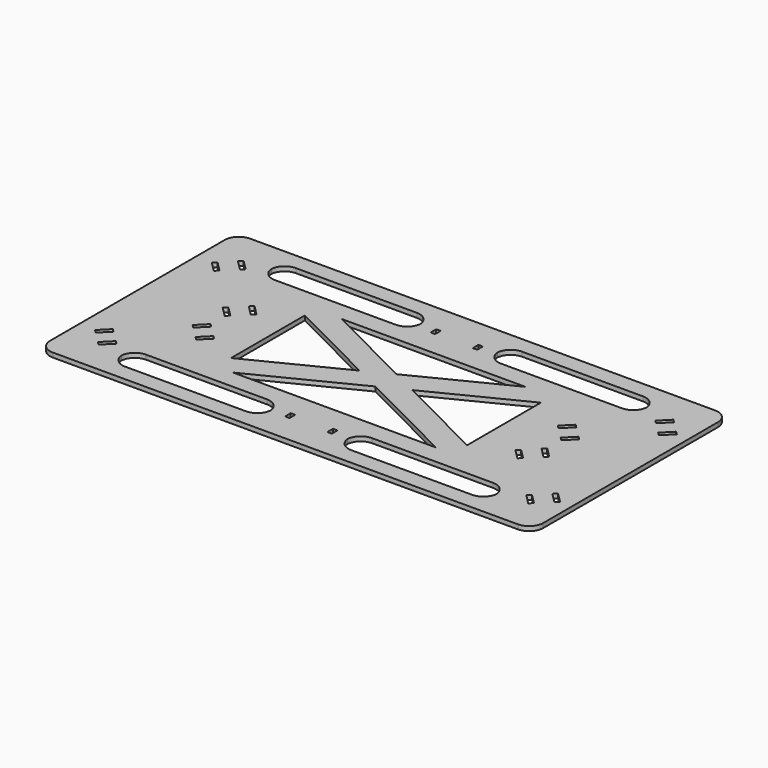
from build123d import *

# Parameters (mm, degrees)
F0_W        = 350
F0_H        = 175
F0_W_2      = 3.175
F0_H_2      = 5
F1_DEPTH    = 3.175
F3_DEPTH    = 25
F4_W        = 105.779197067
F4_H        = 18.4744439814
F5_DEPTH    = 25
F6_T1_DEPTH = 3.175
F6_T3_DEPTH = 53.175
F8_DEPTH    = 25


# Not quite as in the source:
# - a fillet or chamfer that OpenCascade refuses, or shapes differently, is made with other operations: its cross-section is extruded or revolved along the edge and cut away or added


with BuildPart() as f1:
    # F0 (on Top) → F1 (new body)
    with BuildSketch(Plane.XY):
        Rectangle(F0_W, F0_H)
        with Locations((-15, -64.5)):
            Rectangle(F0_W_2, F0_H_2, mode=Mode.SUBTRACT)
        with Locations((15.001, -64.5)):
            Rectangle(F0_W_2, F0_H_2, mode=Mode.SUBTRACT)
        with Locations((-15, 64.5)):
            Rectangle(F0_W_2, F0_H_2, mode=Mode.SUBTRACT)
        with Locations((15.001, 64.5)):
            Rectangle(F0_W_2, F0_H_2, mode=Mode.SUBTRACT)
    extrude(amount=F1_DEPTH)

    # F2 (on face) → F3 (cut)
    with BuildSketch(Plane.XY.offset(3.175)):
        Polygon((-156.5389321881, -44.7351793874), (-163.61, -51.8062471993), (-161.3649359697, -54.0513112295), (-154.2938681579, -46.9802434177), align=None)
        Polygon((-146.2837625406, -54.9903490349), (-153.3548303525, -62.0614168468), (-151.1097663222, -64.3064808771), (-144.0386985103, -57.2354130652), align=None)
        Polygon((159.2439321881, 44.7353613385), (166.315, 51.8064291503), (164.0699359697, 54.0514931806), (156.9988681579, 46.9804253687), align=None)
        Polygon((148.9887625406, 54.990530986), (156.0598303525, 62.0615987979), (153.8147663222, 64.3066628282), (146.7436985103, 57.2355950163), align=None)
        Polygon((-161.3649359697, 54.0513112295), (-163.61, 51.8062471993), (-156.5389321881, 44.7351793874), (-154.2938681579, 46.9802434177), align=None)
        Polygon((-151.0729967696, 64.3432504297), (-153.3180607998, 62.0981863994), (-146.246992988, 55.0271185876), (-144.0019289577, 57.2721826178), align=None)
        Polygon((157.0488681579, -46.9683818087), (164.1199359697, -54.0394496205), (166.365, -51.7943855903), (159.2939321881, -44.7233177784), align=None)
        Polygon((146.7569289577, -57.2603210088), (153.8279967696, -64.3313888207), (156.0730607998, -62.0863247904), (149.001992988, -55.0152569786), align=None)
        Polygon((118.5822592613, -8.5017729121), (125.6533270732, -15.572840724), (127.8983911035, -13.3277766937), (120.8273232916, -6.2567088818), align=None)
        Polygon((108.2903200611, -18.7937121123), (115.361387873, -25.8647799241), (117.6064519033, -23.6197158939), (110.5353840914, -16.548648082), align=None)
        Polygon((120.7773232916, 6.2687524419), (127.8483911035, 13.3398202538), (125.6033270732, 15.5848842841), (118.5322592613, 8.5138164722), align=None)
        Polygon((110.522153644, 16.5239220895), (117.5932214559, 23.5949899013), (115.3481574256, 25.8400539316), (108.2770896138, 18.7689861197), align=None)
        Polygon((-122.8983270732, 15.584702333), (-125.1433911035, 13.3396383027), (-118.0723232916, 6.2685704909), (-115.8272592613, 8.5136345211), align=None)
        Polygon((-112.606387873, 25.8766415332), (-114.8514519033, 23.6315775029), (-107.7803840914, 16.560509691), (-105.5353200611, 18.8055737213), align=None)
        Polygon((-118.0723232916, -6.2685704909), (-125.1433911035, -13.3396383027), (-122.8983270732, -15.584702333), (-115.8272592613, -8.5136345211), align=None)
        Polygon((-107.817153644, -16.5237401384), (-114.8882214559, -23.5948079503), (-112.6431574256, -25.8398719805), (-105.5720896138, -18.7688041687), align=None)
    extrude(amount=-F3_DEPTH, mode=Mode.SUBTRACT)

    # F4 (on face) → F5 (cut)
    with BuildSketch(Plane.XY.offset(3.175)):
        with Locations((-80.2089292556, 66.4726350559)):
            Rectangle(F4_W, F4_H)
        with Locations((-80.2089292556, -66.4726350559)):
            Rectangle(F4_W, F4_H)
        with Locations((80.2089292556, -66.4726350559)):
            Rectangle(F4_W, F4_H)
        with Locations((80.2089292556, 66.4726350559)):
            Rectangle(F4_W, F4_H)
    extrude(amount=-F5_DEPTH, mode=Mode.SUBTRACT)

    # F6: fillet of radius 10 on 20 edges, made by hand

    # F6_s2 → F6_t1 (join)
    with BuildSketch(Plane.XY):
        with BuildLine():
            ThreePointArc((-133.0985277891, -65.7098570466), (-130.169595601, -72.7809248585), (-123.0985277891, -75.7098570466))
            Line((-123.0985277891, -75.7098570466), (-133.0985277891, -75.7098570466))
            Line((-133.0985277891, -75.7098570466), (-133.0985277891, -65.7098570466))
        make_face()
        with BuildLine():
            ThreePointArc((-123.0985277891, -57.2354130652), (-130.169595601, -60.1643452533), (-133.0985277891, -67.2354130652))
            Line((-133.0985277891, -67.2354130652), (-133.0985277891, -57.2354130652))
            Line((-133.0985277891, -57.2354130652), (-123.0985277891, -57.2354130652))
        make_face()
        with BuildLine():
            ThreePointArc((-37.3193307221, -57.2354130652), (-30.2482629102, -60.1643452533), (-27.3193307221, -67.2354130652))
            Line((-27.3193307221, -67.2354130652), (-27.3193307221, -57.2354130652))
            Line((-27.3193307221, -57.2354130652), (-37.3193307221, -57.2354130652))
        make_face()
        with BuildLine():
            ThreePointArc((-37.3193307221, -75.7098570466), (-30.2482629102, -72.7809248585), (-27.3193307221, -65.7098570466))
            Line((-27.3193307221, -65.7098570466), (-27.3193307221, -75.7098570466))
            Line((-27.3193307221, -75.7098570466), (-37.3193307221, -75.7098570466))
        make_face()
        with BuildLine():
            ThreePointArc((123.0985277891, -57.2354130652), (130.169595601, -60.1643452533), (133.0985277891, -67.2354130652))
            Line((133.0985277891, -67.2354130652), (133.0985277891, -57.2354130652))
            Line((133.0985277891, -57.2354130652), (123.0985277891, -57.2354130652))
        make_face()
        with BuildLine():
            ThreePointArc((123.0985277891, -75.7098570466), (130.169595601, -72.7809248585), (133.0985277891, -65.7098570466))
            Line((133.0985277891, -65.7098570466), (133.0985277891, -75.7098570466))
            Line((133.0985277891, -75.7098570466), (123.0985277891, -75.7098570466))
        make_face()
        with BuildLine():
            ThreePointArc((37.3193307221, -57.2354130652), (30.2482629102, -60.1643452533), (27.3193307221, -67.2354130652))
            Line((27.3193307221, -67.2354130652), (27.3193307221, -57.2354130652))
            Line((27.3193307221, -57.2354130652), (37.3193307221, -57.2354130652))
        make_face()
        with BuildLine():
            ThreePointArc((27.3193307221, -65.7098570466), (30.2482629102, -72.7809248585), (37.3193307221, -75.7098570466))
            Line((37.3193307221, -75.7098570466), (27.3193307221, -75.7098570466))
            Line((27.3193307221, -75.7098570466), (27.3193307221, -65.7098570466))
        make_face()
        with BuildLine():
            ThreePointArc((133.0985277891, 65.7098570466), (130.169595601, 72.7809248585), (123.0985277891, 75.7098570466))
            Line((123.0985277891, 75.7098570466), (133.0985277891, 75.7098570466))
            Line((133.0985277891, 75.7098570466), (133.0985277891, 65.7098570466))
        make_face()
        with BuildLine():
            ThreePointArc((133.0985277891, 67.2354130652), (130.169595601, 60.1643452533), (123.0985277891, 57.2354130652))
            Line((123.0985277891, 57.2354130652), (133.0985277891, 57.2354130652))
            Line((133.0985277891, 57.2354130652), (133.0985277891, 67.2354130652))
        make_face()
        with BuildLine():
            ThreePointArc((37.3193307221, 75.7098570466), (30.2482629102, 72.7809248585), (27.3193307221, 65.7098570466))
            Line((27.3193307221, 65.7098570466), (27.3193307221, 75.7098570466))
            Line((27.3193307221, 75.7098570466), (37.3193307221, 75.7098570466))
        make_face()
        with BuildLine():
            ThreePointArc((27.3193307221, 67.2354130652), (30.2482629102, 60.1643452533), (37.3193307221, 57.2354130652))
            Line((37.3193307221, 57.2354130652), (27.3193307221, 57.2354130652))
            Line((27.3193307221, 57.2354130652), (27.3193307221, 67.2354130652))
        make_face()
        with BuildLine():
            ThreePointArc((-27.3193307221, 65.7098570466), (-30.2482629102, 72.7809248585), (-37.3193307221, 75.7098570466))
            Line((-37.3193307221, 75.7098570466), (-27.3193307221, 75.7098570466))
            Line((-27.3193307221, 75.7098570466), (-27.3193307221, 65.7098570466))
        make_face()
        with BuildLine():
            ThreePointArc((-37.3193307221, 57.2354130652), (-30.2482629102, 60.1643452533), (-27.3193307221, 67.2354130652))
            Line((-27.3193307221, 67.2354130652), (-27.3193307221, 57.2354130652))
            Line((-27.3193307221, 57.2354130652), (-37.3193307221, 57.2354130652))
        make_face()
        with BuildLine():
            ThreePointArc((-133.0985277891, 67.2354130652), (-130.169595601, 60.1643452533), (-123.0985277891, 57.2354130652))
            Line((-123.0985277891, 57.2354130652), (-133.0985277891, 57.2354130652))
            Line((-133.0985277891, 57.2354130652), (-133.0985277891, 67.2354130652))
        make_face()
        with BuildLine():
            ThreePointArc((-133.0985277891, 65.7098570466), (-130.169595601, 72.7809248585), (-123.0985277891, 75.7098570466))
            Line((-123.0985277891, 75.7098570466), (-133.0985277891, 75.7098570466))
            Line((-133.0985277891, 75.7098570466), (-133.0985277891, 65.7098570466))
        make_face()
    extrude(amount=F6_T1_DEPTH)

    # F6_s4 → F6_t3 (cut)
    with BuildSketch(Plane.XY.offset(-25)):
        with BuildLine():
            ThreePointArc((-175, 77.5), (-172.0710678119, 84.5710678119), (-165, 87.5))
            Line((-165, 87.5), (-175, 87.5))
            Line((-175, 87.5), (-175, 77.5))
        make_face()
        with BuildLine():
            ThreePointArc((175, 77.5), (172.0710678119, 84.5710678119), (165, 87.5))
            Line((165, 87.5), (175, 87.5))
            Line((175, 87.5), (175, 77.5))
        make_face()
        with BuildLine():
            ThreePointArc((165, -87.5), (172.0710678119, -84.5710678119), (175, -77.5))
            Line((175, -77.5), (175, -87.5))
            Line((175, -87.5), (165, -87.5))
        make_face()
        with BuildLine():
            ThreePointArc((-165, -87.5), (-172.0710678119, -84.5710678119), (-175, -77.5))
            Line((-175, -77.5), (-175, -87.5))
            Line((-175, -87.5), (-165, -87.5))
        make_face()
    extrude(amount=F6_T3_DEPTH, mode=Mode.SUBTRACT)

    # F7 (on face) → F8 (cut)
    with BuildSketch(Plane(origin=(0, 0, 0), x_dir=(1, 0, 0), z_dir=(0, 0, -1))):
        Polygon((83.7561041117, 30.9926522097), (18.7335789211, -1.7076288749), (83.7561041117, -34.4079099596), align=None)
        Polygon((65.1939362288, -43.915361166), (0, -11.1288762757), (-65.1939362288, -43.915361166), align=None)
        Polygon((-18.7335789211, -1.7076288749), (-83.7561041117, 30.9926522097), (-83.7561041117, -34.4079099596), align=None)
        Polygon((71.9849690795, 43.915361166), (-71.9849690795, 43.915361166), (0, 7.7136185258), align=None)
    extrude(amount=-F8_DEPTH, mode=Mode.SUBTRACT)


solid = f1.part
